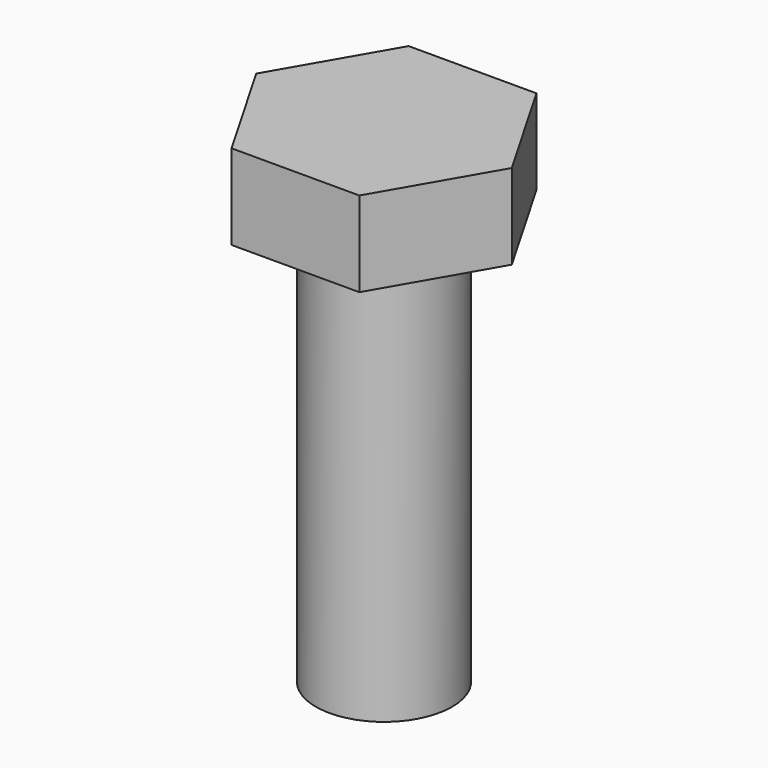
from build123d import *

# Parameters (mm, degrees)
F0_R     = 12.7
F1_DEPTH = 76.2
F3_DEPTH = 15.875


# Not quite as in the source:
# - a feature names something its author has since deleted; it is built from what else it names


with BuildPart() as f1:
    # F0 (on Top) → F1 (new body)
    with BuildSketch(Plane.XY):
        Circle(F0_R)
    extrude(amount=-F1_DEPTH)

    # F2 (on face) → F3 (join)
    with BuildSketch(Plane.XY):
        Polygon((11.9150661804, 20.6375), (-11.9150661804, 20.6375), (-23.8301323608, 0), (-11.9150661804, -20.6375), (11.9150661804, -20.6375), (23.8301323608, 0), align=None)
    extrude(amount=F3_DEPTH)


solid = f1.part
